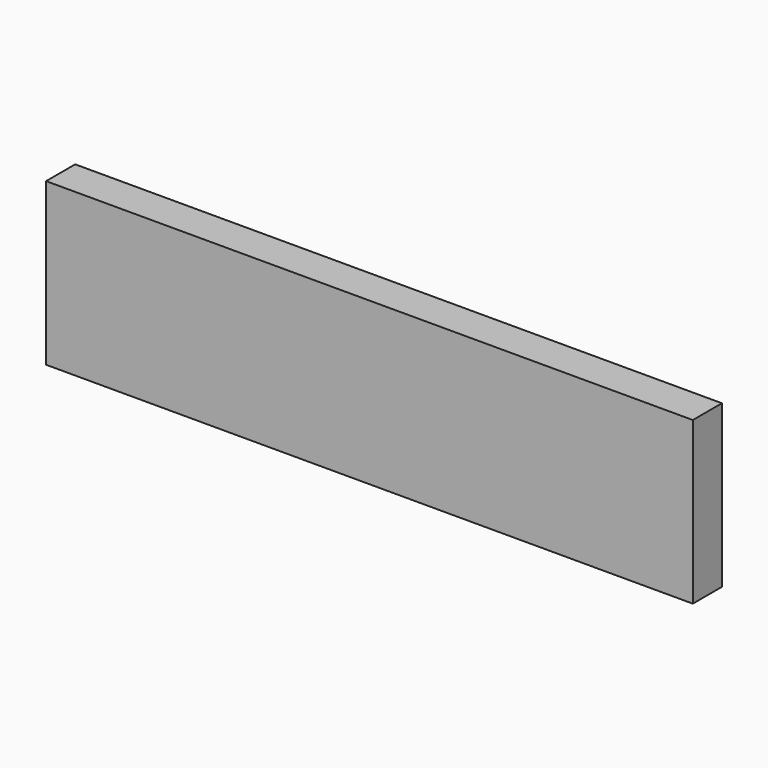
from build123d import *

# Parameters (mm, degrees)
F0_W     = 203.2
F0_H     = 50.8
F1_DEPTH = 6.35
F4_SIZE  = 1.27


# Not quite as in the source:
# - the program builds the solid bodies; features that only make, move or delete a surface that nothing else refers to are left out


with BuildPart() as f1:
    # F0 (on Front) → F1 (new body, symmetric)
    with BuildSketch(Plane.XZ):
        Rectangle(F0_W, F0_H)
    extrude(amount=F1_DEPTH, both=True)

    # F4
    f4_edges = [f1.edges().sort_by_distance(p)[0] for p in [
        (-101.6, 6.35, 0),
        (0, 6.35, -25.4),
        (0, 6.35, 25.4),
        (101.6, 6.35, 0),
    ]]
    chamfer(f4_edges, length=F4_SIZE)


solid = f1.part
